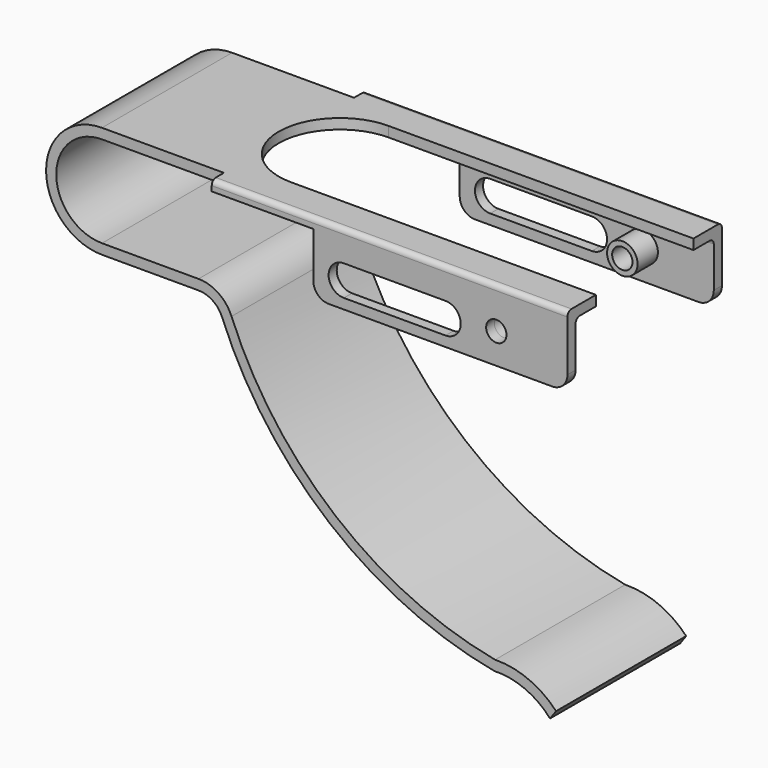
from build123d import *

# Parameters (mm, degrees)
F1_DEPTH  = 16
F2_W      = 70
F2_H      = 3
F3_DEPTH  = 2
F4_W      = 50
F4_H      = 14
F5_DEPTH  = 2
F6_R      = 1
F9_DEPTH  = 2
F11_DEPTH = 38.001
F13_D     = 4
F14_R     = 3
F14_R_2   = 2
F15_DEPTH = 5
F16_R     = 3


# Not quite as in the source:
# - a pattern or mirror of a feature is missing from the dataset's text; its kind, count and spacing are read off the source's solid


with BuildPart() as f1:
    # F0 (on Front) → F1 (new body)
    with BuildSketch(Plane.XZ):
        with BuildLine():
            Line((94, 11), (0, 11))
            ThreePointArc((0, 11), (-11, 0), (0, -11))
            Line((0, -11), (19, -11))
            ThreePointArc((19, -11), (21.7981112342, -11.8562609251), (23.6378571429, -14.1317705916))
            ThreePointArc((23.6378571429, -14.1317705916), (44.801622976, -42.9310620406), (77.2062019292, -58.0057903986))
            ThreePointArc((77.2062019292, -58.0057903986), (83.2137047902, -59.1076967266), (88.1803617021, -62.6624973259))
            Line((88.1803617021, -62.6624973259), (89.3682949555, -61))
            ThreePointArc((89.3682949555, -61), (83.8961627896, -57.2250659611), (77.3621310458, -56))
            ThreePointArc((77.3621310458, -56), (45.985801942, -41.3156371935), (25.493, -13.3844788282))
            ThreePointArc((25.493, -13.3844788282), (22.9173557279, -10.1987652951), (19, -9))
            Line((19, -9), (0, -9))
            ThreePointArc((0, -9), (-9, 0), (0, 9))
            Line((0, 9), (94, 9))
            Line((94, 9), (94, 11))
        make_face()
    extrude(amount=F1_DEPTH)

    # F2 (on face) → F3 (join)
    with BuildSketch(Plane.XY.offset(11)):
        with Locations((59, -17.5)):
            Rectangle(F2_W, F2_H)
    extrude(amount=-F3_DEPTH)

    # F4 (on face) → F5 (join)
    with BuildSketch(Plane.XZ.offset(19)):
        with Locations((69, 4)):
            Rectangle(F4_W, F4_H)
    extrude(amount=-F5_DEPTH)

    # F6
    f6_edges = [f1.edges().sort_by_distance(p)[0] for p in [
        (59, -19, 11),
        (69, -17, 9),
    ]]
    fillet(f6_edges, radius=F6_R)

    # F7: F1 across plane


with BuildPart() as f1_1:
    add(f1.part)
    add(f1.part.mirror(Plane.XZ))

    # F8 (on face) → F9 (cut)
    with BuildSketch(Plane.XY.offset(11)):
        with BuildLine():
            Line((94, 12), (34, 12))
            ThreePointArc((34, 12), (22, 0), (34, -12))
            Line((34, -12), (94, -12))
            Line((94, -12), (94, 12))
        make_face()
    extrude(amount=-F9_DEPTH, mode=Mode.SUBTRACT)

    # F10 (on face) → F11 (cut, through all)
    with BuildSketch(Plane.XZ.offset(19)):
        with BuildLine():
            ThreePointArc((50, 5), (47, 2), (50, -1))
            Line((50, -1), (70, -1))
            ThreePointArc((70, -1), (73, 2), (70, 5))
            Line((70, 5), (50, 5))
        make_face()
    extrude(amount=-F11_DEPTH, mode=Mode.SUBTRACT)

    # F13 (through all)
    with Locations(Plane.XZ.offset(19)):
        with Locations((80, 3)):
            Hole(F13_D / 2)

    # F14 (on face) → F15 (join)
    with BuildSketch(Plane(origin=(0, -17, 0), x_dir=(-1, 0, 0), z_dir=(0, 1, 0))):
        with Locations((-80, 3)):
            Circle(F14_R)
        with Locations((-80, 3)):
            Circle(F14_R_2, mode=Mode.SUBTRACT)
    f15 = extrude(amount=F15_DEPTH)

    # F15_copies: F15 across plane
    add(f15.mirror(Plane.ZX))

    # F16
    f16_edges = [f1_1.edges().sort_by_distance(p)[0] for p in [
        (44, -18, -3),
        (44, 18, -3),
        (94, -18, -3),
        (94, 18, -3),
    ]]
    fillet(f16_edges, radius=F16_R)


solid = f1_1.part
